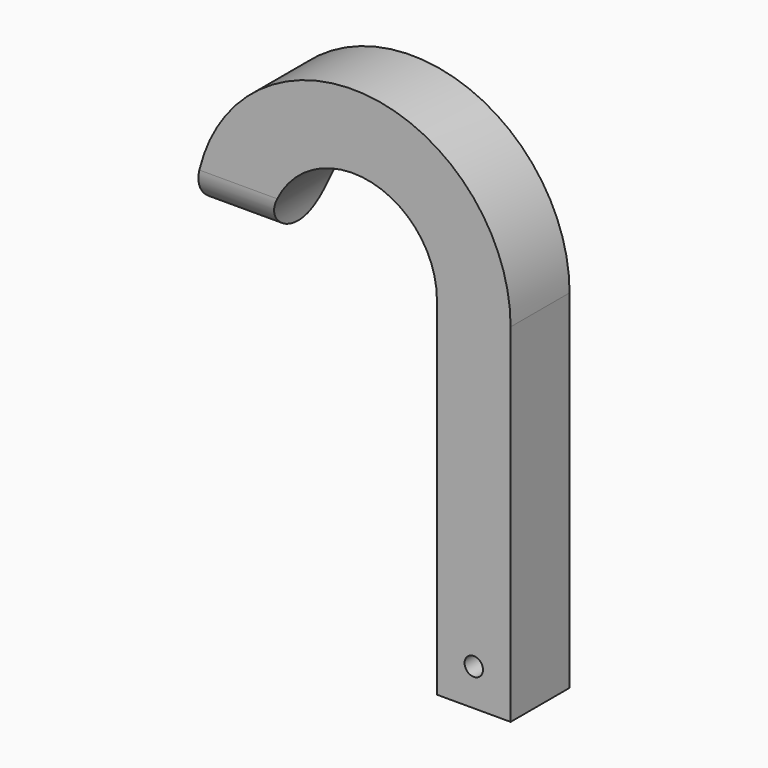
from build123d import *

# Parameters (mm, degrees)
F0_R     = 3.175
F1_DEPTH = 25.4
F2_R     = 12.7
F3_R     = 12.69999


# Not quite as in the source:
# - a fillet or chamfer is up to 0.001 mm smaller than in the source, because OpenCascade refuses the exact size


with BuildPart() as f1:
    # F0 (on Front) → F1 (new body)
    with BuildSketch(Plane.XZ):
        with BuildLine():
            Line((0, 44.897188701), (0, -74.9478926185))
            Line((0, -74.9478926185), (25.4, -74.9478926185))
            Line((25.4, -74.9478926185), (25.4, 44.897188701))
            ThreePointArc((25.4, 44.897188701), (-28.9774724535, 99.2746611545), (-83.3549449071, 44.897188701))
            Line((-83.3549449071, 44.897188701), (-57.9549449071, 44.897188701))
            ThreePointArc((-57.9549449071, 44.897188701), (-28.9774724535, 73.8746611545), (0, 44.897188701))
        make_face()
        with Locations((12.7, -62.2478926185)):
            Circle(F0_R, mode=Mode.SUBTRACT)
    extrude(amount=F1_DEPTH)

    # F2
    f2_edges = [f1.edges().sort_by_distance(p)[0] for p in [
        (-70.654945, -25.4, 44.897189),
    ]]
    fillet(f2_edges, radius=F2_R)

    # F3 (radius 12.7 in the source; OpenCascade refuses exactly that, so slightly less here)
    f3_edges = [f1.edges().sort_by_distance(p)[0] for p in [
        (-70.654945, 0, 44.897189),
    ]]
    fillet(f3_edges, radius=F3_R)


solid = f1.part
